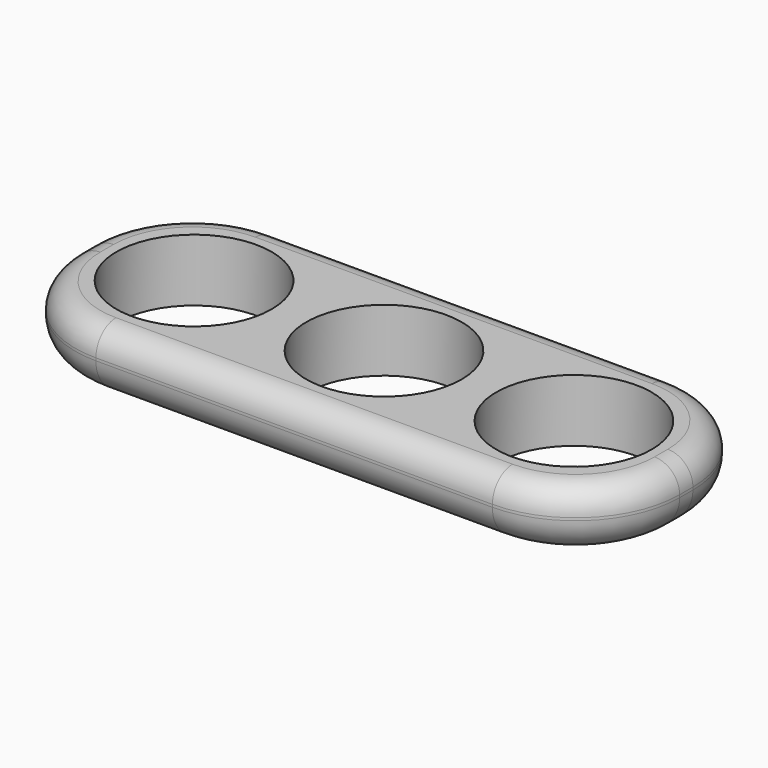
from build123d import *

# Parameters (mm, degrees)
F0_R     = 11.2
F1_DEPTH = 9
F2_R     = 3.6213203436
F3_R     = 4.99999


# Not quite as in the source:
# - a fillet or chamfer is up to 0.001 mm smaller than in the source, because OpenCascade refuses the exact size


with BuildPart() as f1:
    # F0 (on Top) → F1 (new body)
    with BuildSketch(Plane.XY):
        with BuildLine():
            Line((28.6, 16.2), (-28.6, 16.2))
            ThreePointArc((-28.6, 16.2), (-39.2066017178, 11.8066017178), (-43.6, 1.2))
            Line((-43.6, 1.2), (-43.6, -1.2))
            ThreePointArc((-43.6, -1.2), (-39.2066017178, -11.8066017178), (-28.6, -16.2))
            Line((-28.6, -16.2), (28.6, -16.2))
            ThreePointArc((28.6, -16.2), (39.2066017178, -11.8066017178), (43.6, -1.2))
            Line((43.6, -1.2), (43.6, 1.2))
            ThreePointArc((43.6, 1.2), (39.2066017178, 11.8066017178), (28.6, 16.2))
        make_face()
        with Locations((-27.4, 0)):
            Circle(F0_R, mode=Mode.SUBTRACT)
        Circle(F0_R, mode=Mode.SUBTRACT)
        with Locations((27.4, 0)):
            Circle(F0_R, mode=Mode.SUBTRACT)
    extrude(amount=F1_DEPTH)

    # F2
    f2_edges = [f1.edges().sort_by_distance(p)[0] for p in [
        (39.206602, 11.806602, 9),
    ]]
    fillet(f2_edges, radius=F2_R)

    # F3 (radius 5 in the source; OpenCascade refuses exactly that, so slightly less here)
    f3_edges = [f1.edges().sort_by_distance(p)[0] for p in [
        (0, 16.2, 0),
        (39.206602, 11.806602, 0),
    ]]
    fillet(f3_edges, radius=F3_R)


solid = f1.part
